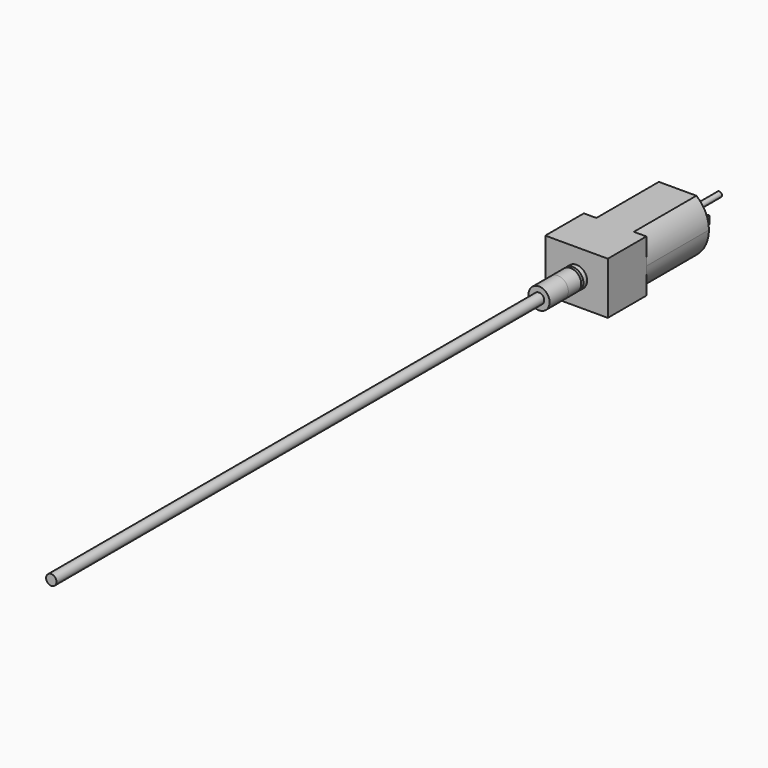
from build123d import *

# Parameters (mm, degrees)
F0_W      = 24.25
F0_H      = 10
F1_DEPTH  = 6
F3_DEPTH  = 15
F4_R      = 2.025
F5_DEPTH  = 4.5
F6_R      = 2.025
F6_R_2    = 1.5
F7_DEPTH  = 3.6
F9_DEPTH  = 3.6
F10_R     = 2.5
F11_DEPTH = 1.2
F12_W     = 0.35
F12_H     = 1.5
F13_DEPTH = 2.6
F14_R     = 0.5
F15_DEPTH = 8.8
F16_R     = 2.025
F17_DEPTH = 3.1
F18_R     = 2.025
F19_DEPTH = 4.5
F20_R     = 1
F21_DEPTH = 3
F22_DEPTH = 120


with BuildPart() as f1:
    # F0 (on Right) → F1 (new body, symmetric)
    with BuildSketch(Plane.YZ):
        Rectangle(F0_W, F0_H)
    extrude(amount=F1_DEPTH, both=True)

    # F2 (on face) → F3 (cut)
    with BuildSketch(Plane(origin=(0, 12.125, 0), x_dir=(-1, 0, 0), z_dir=(0, 1, 0))):
        with BuildLine():
            ThreePointArc((-3.6, -5), (-5.3689269262, -2.7730849257), (-6, -2.1e-09))
            Line((-6, -2.1e-09), (-6, -5))
            Line((-6, -5), (-3.6, -5))
        make_face()
        with BuildLine():
            ThreePointArc((-6, -2.1e-09), (-5.3689269271, 2.7730849238), (-3.6, 5))
            Line((-3.6, 5), (-6, 5))
            Line((-6, 5), (-6, -2.1e-09))
        make_face()
        with BuildLine():
            ThreePointArc((3.6, 5), (5.3689269271, 2.7730849238), (6, -2.1e-09))
            Line((6, -2.1e-09), (6, 5))
            Line((6, 5), (3.6, 5))
        make_face()
        with BuildLine():
            Line((3.6, -5), (6, -5))
            Line((6, -5), (6, -2.1e-09))
            ThreePointArc((6, -2.1e-09), (5.3689269262, -2.7730849257), (3.6, -5))
        make_face()
    extrude(amount=-F3_DEPTH, mode=Mode.SUBTRACT)

    # F4 (on face) → F5 (join)
    with BuildSketch(Plane.XZ.offset(12.125)):
        Circle(F4_R)
    extrude(amount=F5_DEPTH)

    # F6 (on face) → F7 (cut)
    with BuildSketch(Plane.XZ.offset(16.625)):
        Circle(F6_R)
        Circle(F6_R_2, mode=Mode.SUBTRACT)
    extrude(amount=-F7_DEPTH, mode=Mode.SUBTRACT)

    # F8 (on face) → F9 (cut, through all)
    with BuildSketch(Plane.XZ.offset(16.625)):
        with BuildLine():
            ThreePointArc((1.1180339887, 1), (0, 1.5), (-1.1180339887, 1))
            Line((-1.1180339887, 1), (1.1180339887, 1))
        make_face()
    extrude(amount=-F9_DEPTH, mode=Mode.SUBTRACT)

    # F10 (on face) → F11 (join)
    with BuildSketch(Plane(origin=(0, 12.125, 0), x_dir=(-1, 0, 0), z_dir=(0, 1, 0))):
        Circle(F10_R)
    extrude(amount=F11_DEPTH)

    # F12 (on face) → F13 (join)
    with BuildSketch(Plane(origin=(0, 12.125, 0), x_dir=(-1, 0, 0), z_dir=(0, 1, 0))):
        with Locations((-3.825, 0)):
            Rectangle(F12_W, F12_H)
        with Locations((3.825, 0)):
            Rectangle(F12_W, F12_H)
    extrude(amount=F13_DEPTH)

    # F14 (on face) → F15 (join)
    with BuildSketch(Plane(origin=(0, 13.325, 0), x_dir=(-1, 0, 0), z_dir=(0, 1, 0))):
        Circle(F14_R)
    extrude(amount=F15_DEPTH)


with BuildPart() as f17:
    # F16 (on face) → F17 (new body)
    with BuildSketch(Plane.XZ.offset(16.625)):
        Circle(F16_R)
        with BuildLine():
            ThreePointArc((1.1180339887, 1), (0, -1.5), (-1.1180339887, 1))
            Line((-1.1180339887, 1), (1.1180339887, 1))
        make_face(mode=Mode.SUBTRACT)
    extrude(amount=-F17_DEPTH)

    # F18 (on face) → F19 (join)
    with BuildSketch(Plane.XZ.offset(16.625)):
        Circle(F18_R)
    extrude(amount=F19_DEPTH)

    # F20 (on face) → F21 (cut)
    with BuildSketch(Plane.XZ.offset(21.125)):
        Circle(F20_R)
    extrude(amount=-F21_DEPTH, mode=Mode.SUBTRACT)


with BuildPart() as f22:
    # F22 (new): a face of the model
    f22_faces = [f17.part.faces().sort_by_distance(p)[0] for p in [
        (0, -18.125, 0),
    ]]
    extrude(f22_faces, amount=F22_DEPTH)


solid = Compound([f1.part, f17.part, f22.part])
